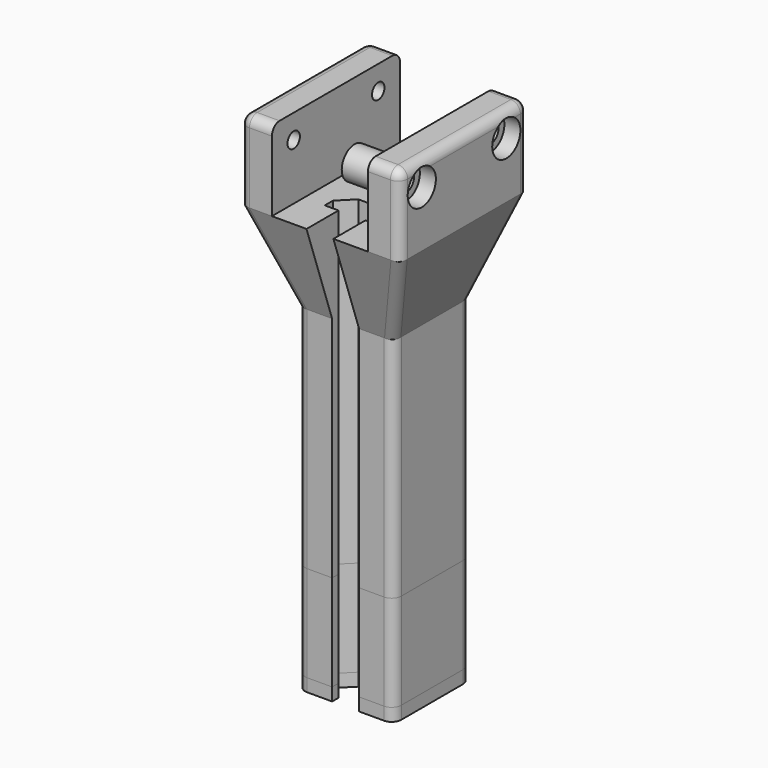
from build123d import *

# Parameters (mm, degrees)
F0_R          = 1.5
F1_DEPTH      = 100
F2_W          = 10
F2_H          = 25
F3_DEPTH      = 30
F4_DEPTH      = 10
F5_DEPTH      = 10
F7_DEPTH      = 132
F8_DEPTH      = 110
F9_F1_R       = 3
F9_F2_R       = 3
F9_F3_R       = 3
F9_F4_R       = 3
F9_F5_R       = 3
F9_F6_R       = 3
F9_F7_R       = 3
F9_F8_R       = 3
F9_F9_R       = 3
F9_F10_R      = 3
F9_F11_R      = 3
F9_F12_R      = 3
F10_R         = 3.25
F11_DEPTH     = 15
F12_R         = 2.425
F13_DEPTH     = 80
F14_R         = 5.5
F15_DEPTH     = 5
F17_DEPTH     = 124
F18_W         = 8.4
F18_H         = 10
F19_DEPTH     = 30
F20_DEPTH     = 30
F21_T1_DEPTH  = 14.5
F21_T3_DEPTH  = 14.5
F21_T5_DEPTH  = 44
F21_T8_ANGLE  = 90
F21_T10_ANGLE = 90
F21_T12_ANGLE = 90
F21_T14_ANGLE = 90
F22_R         = 5
F22_R_2       = 3.5
F23_DEPTH     = 11
F24_DEPTH     = 4


# Not quite as in the source:
# - a fillet or chamfer that OpenCascade refuses, or shapes differently, is made with other operations: its cross-section is extruded or revolved along the edge and cut away or added


with BuildPart() as f1:
    # F0 (on Top) → F1 (new body)
    with BuildSketch(Plane.XY):
        Polygon((-12, -15), (12, -15), (15, -15), (15, -12), (15, 12), (15, 15), (12, 15), (-12, 15), (-15, 15), (-15, 12), (-15, -12), (-15, -15), align=None)
        Circle(F0_R, mode=Mode.SUBTRACT)
    extrude(amount=F1_DEPTH)

    # F2 (on face) → F3 (join, through all)
    with BuildSketch(Plane.XZ.offset(15)):
        with Locations((20, 112.5)):
            Rectangle(F2_W, F2_H)
        Polygon((25, 100), (15, 100), (15, 71.2687671185), align=None)
        Polygon((-15, 71.2687671185), (-15, 100), (-25, 100), align=None)
        with Locations((-20, 112.5)):
            Rectangle(F2_W, F2_H)
    extrude(amount=-F3_DEPTH)

    # F4 (add): faces of the model
    f4_faces = [f1.faces().sort_by_distance(p)[0] for p in [
        (0, -15, 61.3177895676),
        (0, -15, 61.3177895676),
    ]]
    extrude(f4_faces, amount=F4_DEPTH)

    # F5 (add): faces of the model
    f5_faces = [f1.faces().sort_by_distance(p)[0] for p in [
        (0, 15, 61.3177895676),
        (0, 15, 61.3177895676),
    ]]
    extrude(f5_faces, amount=F5_DEPTH)

    # F6 (on face) → F7 (cut)
    with BuildSketch(Plane(origin=(-25, 0, 0), x_dir=(0, -1, 0), z_dir=(-1, 0, 0))):
        Polygon((25, 100), (15, 71.2687671185), (25, 71.2687671185), align=None)
        Polygon((-25, 71.2687671185), (-15, 71.2687671185), (-25, 100), align=None)
    extrude(amount=-F7_DEPTH, mode=Mode.SUBTRACT)

    # F8 (cut): faces of the model
    f8_faces = [f1.faces().sort_by_distance(p)[0] for p in [
        (0, -20, 71.2687671185),
        (0, 20, 71.2687671185),
    ]]
    extrude(f8_faces, amount=-F8_DEPTH, mode=Mode.SUBTRACT)

    # F9: fillet of radius 3 on 12 edges, made by hand

    # F9_f1
    f9_f1_edges = [f1.edges().sort_by_distance(p)[0] for p in [
        (25, 25, 112.5),
    ]]
    fillet(f9_f1_edges, radius=F9_F1_R)

    # F9_f2
    f9_f2_edges = [f1.edges().sort_by_distance(p)[0] for p in [
        (25, -25, 112.5),
    ]]
    fillet(f9_f2_edges, radius=F9_F2_R)

    # F9_f3
    f9_f3_edges = [f1.edges().sort_by_distance(p)[0] for p in [
        (-25, -25, 112.5),
    ]]
    fillet(f9_f3_edges, radius=F9_F3_R)

    # F9_f4
    f9_f4_edges = [f1.edges().sort_by_distance(p)[0] for p in [
        (-25, 25, 112.5),
    ]]
    fillet(f9_f4_edges, radius=F9_F4_R)

    # F9_f5
    f9_f5_edges = [f1.edges().sort_by_distance(p)[0] for p in [
        (19.5606601718, -19.5606601718, 84.3721060674),
    ]]
    fillet(f9_f5_edges, radius=F9_F5_R)

    # F9_f6
    f9_f6_edges = [f1.edges().sort_by_distance(p)[0] for p in [
        (19.5606601718, 19.5606601718, 84.3721060674),
    ]]
    fillet(f9_f6_edges, radius=F9_F6_R)

    # F9_f7
    f9_f7_edges = [f1.edges().sort_by_distance(p)[0] for p in [
        (-19.5606601718, -19.5606601718, 84.3721060674),
    ]]
    fillet(f9_f7_edges, radius=F9_F7_R)

    # F9_f8
    f9_f8_edges = [f1.edges().sort_by_distance(p)[0] for p in [
        (-19.5606601718, 19.5606601718, 84.3721060674),
    ]]
    fillet(f9_f8_edges, radius=F9_F8_R)

    # F9_f9
    f9_f9_edges = [f1.edges().sort_by_distance(p)[0] for p in [
        (15, 15, 36.8010775644),
    ]]
    fillet(f9_f9_edges, radius=F9_F9_R)

    # F9_f10
    f9_f10_edges = [f1.edges().sort_by_distance(p)[0] for p in [
        (15, -15, 36.8010775644),
    ]]
    fillet(f9_f10_edges, radius=F9_F10_R)

    # F9_f11
    f9_f11_edges = [f1.edges().sort_by_distance(p)[0] for p in [
        (-15, -15, 36.8010775644),
    ]]
    fillet(f9_f11_edges, radius=F9_F11_R)

    # F9_f12
    f9_f12_edges = [f1.edges().sort_by_distance(p)[0] for p in [
        (-15, 15, 36.8010775644),
    ]]
    fillet(f9_f12_edges, radius=F9_F12_R)

    # F10 (on face) → F11 (cut, symmetric)
    with BuildSketch(Plane(origin=(15, 0, 0), x_dir=(0, -1, 0), z_dir=(-1, 0, 0))):
        with Locations((-16.5, 117.5)):
            Circle(F10_R)
        with Locations((16.5, 117.5)):
            Circle(F10_R)
    extrude(amount=F11_DEPTH, both=True, mode=Mode.SUBTRACT)

    # F12 (on face) → F13 (cut)
    with BuildSketch(Plane.YZ.offset(25)):
        with Locations((16.5, 117.5)):
            Circle(F12_R)
        with Locations((-16.5, 117.5)):
            Circle(F12_R)
    extrude(amount=-F13_DEPTH, mode=Mode.SUBTRACT)

    # F14 (on face) → F15 (cut)
    with BuildSketch(Plane.YZ.offset(25)):
        with Locations((-16.5, 117.5)):
            Circle(F14_R)
        with Locations((16.5, 117.5)):
            Circle(F14_R)
    extrude(amount=-F15_DEPTH, mode=Mode.SUBTRACT)

    # F16 (on face) → F17 (cut)
    with BuildSketch(Plane(origin=(0, 0, 0), x_dir=(1, 0, 0), z_dir=(0, 0, -1))):
        Polygon((4.2, 15), (0, 15), (-4.2, 15), (-4.2, 12.5), (-8.5, 12.5), (-8.5, 9.3), (-4.1, 4.9), (0, 4.9), (4.1, 4.9), (8.5, 9.3), (8.5, 12.5), (4.2, 12.5), align=None)
        Polygon((-4.2, -12.5), (-4.2, -15), (0, -15), (4.2, -15), (4.2, -12.5), (8.5, -12.5), (8.5, -9.3), (4.1, -4.9), (0, -4.9), (-4.1, -4.9), (-8.5, -9.3), (-8.5, -12.5), align=None)
    extrude(amount=-F17_DEPTH, mode=Mode.SUBTRACT)

    # F18 (on face) → F19 (cut)
    with BuildSketch(Plane.XY.offset(100)):
        with Locations((0, 20)):
            Rectangle(F18_W, F18_H)
        with Locations((0, -20)):
            Rectangle(F18_W, F18_H)
    extrude(amount=-F19_DEPTH, mode=Mode.SUBTRACT)

    # F20 (add): a face of the model
    f20_faces = [f1.faces().sort_by_distance(p)[0] for p in [
        (-13.8213203436, 13.8213203436, 0),
    ]]
    extrude(f20_faces, amount=F20_DEPTH)

    # F21: fillet of radius 3 on 10 edges, made by hand

    # F21_s2 → F21_t1 (cut)
    with BuildSketch(Plane.YZ.offset(-22)):
        with BuildLine():
            ThreePointArc((-22, 125), (-24.1213203436, 124.1213203436), (-25, 122))
            Line((-25, 122), (-25, 125))
            Line((-25, 125), (-22, 125))
        make_face()
        with BuildLine():
            ThreePointArc((25, 122), (24.1213203436, 124.1213203436), (22, 125))
            Line((22, 125), (25, 125))
            Line((25, 125), (25, 122))
        make_face()
    extrude(amount=F21_T1_DEPTH, mode=Mode.SUBTRACT)

    # F21_s4 → F21_t3 (cut)
    with BuildSketch(Plane.YZ.offset(7.5)):
        with BuildLine():
            ThreePointArc((-25, 122), (-24.1213203436, 124.1213203436), (-22, 125))
            Line((-22, 125), (-25, 125))
            Line((-25, 125), (-25, 122))
        make_face()
        with BuildLine():
            ThreePointArc((25, 122), (24.1213203436, 124.1213203436), (22, 125))
            Line((22, 125), (25, 125))
            Line((25, 125), (25, 122))
        make_face()
    extrude(amount=F21_T3_DEPTH, mode=Mode.SUBTRACT)

    # F21_s6 → F21_t5 (cut)
    with BuildSketch(Plane.XZ.offset(-22)):
        with BuildLine():
            ThreePointArc((-25, 122), (-24.1213203436, 124.1213203436), (-22, 125))
            Line((-22, 125), (-25, 125))
            Line((-25, 125), (-25, 122))
        make_face()
        with BuildLine():
            ThreePointArc((22, 125), (24.1213203436, 124.1213203436), (25, 122))
            Line((25, 122), (25, 125))
            Line((25, 125), (22, 125))
        make_face()
    extrude(amount=F21_T5_DEPTH, mode=Mode.SUBTRACT)

    # F21_s7 → F21_t8 (revolve, cut)
    with BuildSketch(Plane.YZ.offset(-22)):
        with BuildLine():
            ThreePointArc((-25, 122), (-24.1213203436, 124.1213203436), (-22, 125))
            Line((-22, 125), (-25, 125))
            Line((-25, 125), (-25, 122))
        make_face()
    revolve(axis=Axis((-22, -22, 125), (0, 0, -1)), revolution_arc=F21_T8_ANGLE, mode=Mode.SUBTRACT)

    # F21_s9 → F21_t10 (revolve, cut)
    with BuildSketch(Plane.XZ.offset(-22)):
        with BuildLine():
            ThreePointArc((-25, 122), (-24.1213203436, 124.1213203436), (-22, 125))
            Line((-22, 125), (-25, 125))
            Line((-25, 125), (-25, 122))
        make_face()
    revolve(axis=Axis((-22, 22, 125), (0, 0, -1)), revolution_arc=F21_T10_ANGLE, mode=Mode.SUBTRACT)

    # F21_s11 → F21_t12 (revolve, cut)
    with BuildSketch(Plane.XZ.offset(22)):
        with BuildLine():
            ThreePointArc((25, 122), (24.1213203436, 124.1213203436), (22, 125))
            Line((22, 125), (25, 125))
            Line((25, 125), (25, 122))
        make_face()
    revolve(axis=Axis((22, -22, 125), (0, 0, -1)), revolution_arc=F21_T12_ANGLE, mode=Mode.SUBTRACT)

    # F21_s13 → F21_t14 (revolve, cut)
    with BuildSketch(Plane.XZ.offset(-22)):
        with BuildLine():
            ThreePointArc((25, 122), (24.1213203436, 124.1213203436), (22, 125))
            Line((22, 125), (25, 125))
            Line((25, 125), (25, 122))
        make_face()
    revolve(axis=Axis((22, 22, 125), (0, 0, 1)), revolution_arc=F21_T14_ANGLE, mode=Mode.SUBTRACT)


with BuildPart() as f23:
    # F22 (on face) → F23 (new body)
    with BuildSketch(Plane(origin=(15, 0, 0), x_dir=(0, -1, 0), z_dir=(-1, 0, 0))):
        with Locations((16.5, 117.5)):
            Circle(F22_R)
        with Locations((16.5, 117.5)):
            Circle(F22_R_2, mode=Mode.SUBTRACT)
    extrude(amount=F23_DEPTH)


with BuildPart() as f24:
    # F24 (new): a face of the model
    f24_faces = [f1.part.faces().sort_by_distance(p)[0] for p in [
        (-13.8213203436, 13.8213203436, -30),
    ]]
    extrude(f24_faces, amount=F24_DEPTH)


solid = Compound([f1.part, f23.part, f24.part])
